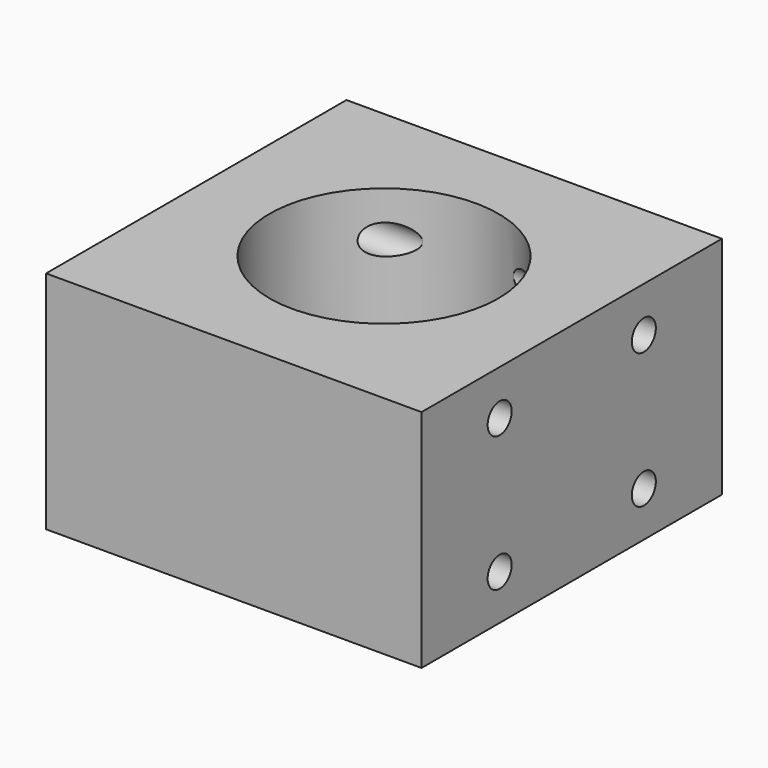
from build123d import *

# Parameters (mm, degrees)
F0_W     = 50
F0_H     = 30
F0_R     = 2
F1_DEPTH = 25
F2_R     = 15.25
F3_DEPTH = 30.001


# Not quite as in the source:
# - a feature names something its author has since deleted; it is built from what else it names


with BuildPart() as f1:
    # F0 (on Right) → F1 (new body, symmetric)
    with BuildSketch(Plane.YZ):
        Rectangle(F0_W, F0_H)
        with Locations((-12.0000001043, -9)):
            Circle(F0_R, mode=Mode.SUBTRACT)
        with Locations((12.0000001043, -9)):
            Circle(F0_R, mode=Mode.SUBTRACT)
        with Locations((-12, 9)):
            Circle(F0_R, mode=Mode.SUBTRACT)
        with Locations((12, 9)):
            Circle(F0_R, mode=Mode.SUBTRACT)
    extrude(amount=F1_DEPTH, both=True)

    # F2 (on face) → F3 (cut, through all)
    with BuildSketch(Plane.XY.offset(15)):
        Circle(F2_R)
    extrude(amount=-F3_DEPTH, mode=Mode.SUBTRACT)


solid = f1.part
